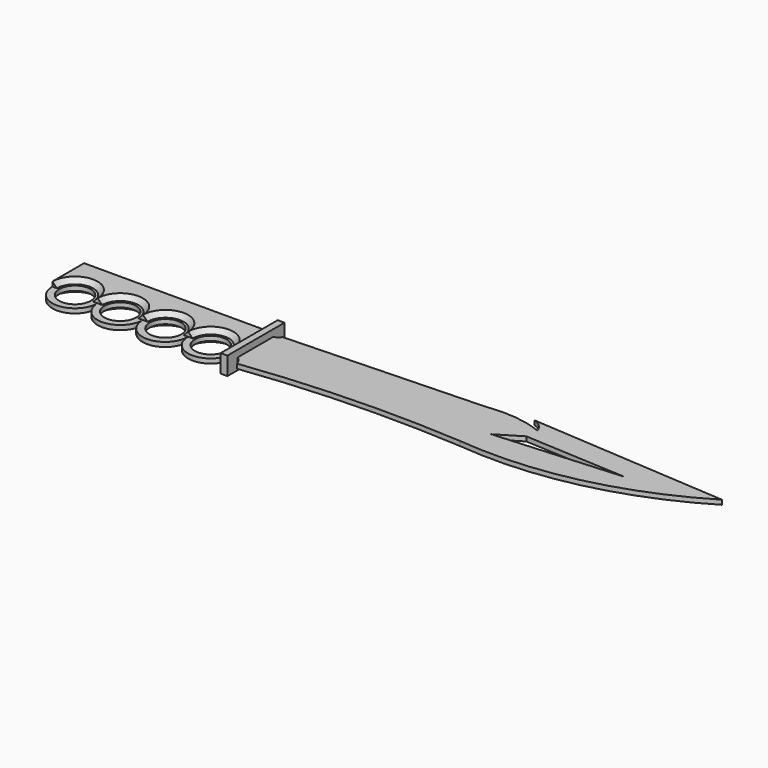
from build123d import *

# Parameters (mm, degrees)
F0_R          = 8.89
F1_DEPTH      = 2.54
F3_DEPTH      = 25.4
F5_DEPTH      = 2.54
F7_DEPTH      = 2.54
F8_T2_ANGLE   = 306.5001793885
F8_T4_ANGLE   = 306.5001793885
F8_T6_ANGLE   = 306.5001793885
F8_T8_ANGLE   = 306.5001793885
F8_2_T2_ANGLE = 306.5001793885
F8_2_T4_ANGLE = 306.5001793885
F8_2_T6_ANGLE = 306.5001793885
F8_2_T8_ANGLE = 306.5001793885
F10_DEPTH     = 3.81


# Not quite as in the source:
# - a fillet or chamfer that OpenCascade refuses, or shapes differently, is made with other operations: its cross-section is extruded or revolved along the edge and cut away or added


with BuildPart() as f1:
    # F0 (on Top) → F1 (new body)
    with BuildSketch(Plane.XY):
        with BuildLine():
            Line((0, 22.2569602452), (0, 0))
            ThreePointArc((0, 0), (4.5429449248, -2.2524889562), (7.2743112207, -6.5246890036))
            ThreePointArc((7.2743112207, -6.5246890036), (68.2558827077, -1.7283700883), (129.4168248237, -2.7752204279))
            ThreePointArc((129.4168248237, -2.7752204279), (193.990196572, 1.2229597331), (254, 25.4))
            Line((254, 25.4), (142.8799988323, 32.9367792524))
            Line((142.8799988323, 32.9367792524), (119.2322895651, 29.7860647099))
            ThreePointArc((119.2322895651, 29.7860647099), (116.0841208365, 29.5940132977), (112.9331847352, 29.4545436828))
            Line((112.9331847352, 29.4545436828), (7.2743112207, 25.6611633832))
            ThreePointArc((7.2743112207, 25.6611633832), (4.0157254245, 23.1501104869), (0, 22.2569602452))
        make_face()
        with BuildLine():
            ThreePointArc((-25.3981255835, -0.218189517), (-12.5909012159, -12.6995313872), (0, 0))
            Line((0, 0), (0, 22.2569602452))
            Line((0, 22.2569602452), (-34.8408528237, 22.2569602452))
            ThreePointArc((-34.8408528237, 22.2569602452), (-50.8, 21.91440634), (-66.7591471763, 22.2569602452))
            Line((-66.7591471763, 22.2569602452), (-101.6, 22.2569602452))
            Line((-101.6, 22.2569602452), (-101.6, 0))
            ThreePointArc((-101.6, 0), (-88.9, -12.7), (-76.2, 0))
            ThreePointArc((-76.2, 0), (-63.6090987841, -12.6995313872), (-50.8018744165, -0.218189517))
            ThreePointArc((-50.8018744165, -0.218189517), (-38.1, -12.9200800362), (-25.3981255835, -0.218189517))
        make_face()
        with Locations((-88.9, 0)):
            Circle(F0_R, mode=Mode.SUBTRACT)
        with Locations((-63.5, 0)):
            Circle(F0_R, mode=Mode.SUBTRACT)
        with BuildLine():
            ThreePointArc((-50.8, 0), (-50.8004686128, -0.1090987841), (-50.8018744165, -0.218189517))
            ThreePointArc((-50.8018744165, -0.218189517), (-50.8014057346, -0.1090907335), (-50.8, 0))
        make_face(mode=Mode.SUBTRACT)
        with Locations((-38.1, 0)):
            Circle(F0_R, mode=Mode.SUBTRACT)
        with BuildLine():
            ThreePointArc((-25.4, 0), (-25.3985942654, -0.1090907335), (-25.3981255835, -0.218189517))
            ThreePointArc((-25.3981255835, -0.218189517), (-25.3995313872, -0.1090987841), (-25.4, 0))
        make_face(mode=Mode.SUBTRACT)
        with Locations((-12.7, 0)):
            Circle(F0_R, mode=Mode.SUBTRACT)
        with BuildLine():
            ThreePointArc((-66.7591471763, 22.2569602452), (-50.8, 21.91440634), (-34.8408528237, 22.2569602452))
            Line((-34.8408528237, 22.2569602452), (-66.7591471763, 22.2569602452))
        make_face()
        with BuildLine():
            ThreePointArc((-50.8, 0), (-50.8014057346, -0.1090907335), (-50.8018744165, -0.218189517))
            ThreePointArc((-50.8018744165, -0.218189517), (-50.8004686128, -0.1090987841), (-50.8, 0))
        make_face()
        with BuildLine():
            ThreePointArc((-25.4, 0), (-25.3995313872, -0.1090987841), (-25.3981255835, -0.218189517))
            ThreePointArc((-25.3981255835, -0.218189517), (-25.3985942654, -0.1090907335), (-25.4, 0))
        make_face()
    extrude(amount=F1_DEPTH)

    # F2 (on face) → F3 (cut)
    with BuildSketch(Plane.XY.offset(2.54)):
        with BuildLine():
            ThreePointArc((119.2322895651, 29.7860647099), (134.7574672595, 29.9044998636), (149.8305946589, 26.1834785342))
            ThreePointArc((149.8305946589, 26.1834785342), (147.1610546869, 30.3894267459), (142.8799988323, 32.9367792524))
            Line((142.8799988323, 32.9367792524), (119.2322895651, 29.7860647099))
        make_face()
        Polygon((207.085609436, 15.6457461417), (149.4793444872, 18.8070647418), (136.1315399408, 10.7281366363), align=None)
    extrude(amount=-F3_DEPTH, mode=Mode.SUBTRACT)


with BuildPart() as f5:
    # F4 (on face) → F5 (new body)
    with BuildSketch(Plane.XY.offset(2.54)):
        with BuildLine():
            Line((0, 0), (0, 22.2569602452))
            Line((0, 22.2569602452), (-101.6, 22.2569602452))
            Line((-101.6, 22.2569602452), (-101.6, 0))
            Line((-101.6, 0), (-97.79, 0))
            ThreePointArc((-97.79, 0), (-88.9, 8.89), (-80.01, 0))
            Line((-80.01, 0), (-76.2, 0))
            Line((-76.2, 0), (-72.39, 0))
            ThreePointArc((-72.39, 0), (-63.5, 8.89), (-54.61, 0))
            Line((-54.61, 0), (-46.99, 0))
            ThreePointArc((-46.99, 0), (-38.1, 8.89), (-29.21, 0))
            Line((-29.21, 0), (-21.59, 0))
            ThreePointArc((-21.59, 0), (-12.7, 8.89), (-3.81, 0))
            Line((-3.81, 0), (0, 0))
        make_face()
    extrude(amount=F5_DEPTH)

    # F8: chamfer of 3.81 on 4 edges, made by hand

    # F8_s1 → F8_t2 (revolve, cut)
    with BuildSketch(Plane(origin=(-70.8899847432, 35.7313546731, 0), x_dir=(0, 0, 1), z_dir=(0.892979648, -0.4500970431, 0))):
        Polygon((5.08, 52.7136271329), (1.27, 48.9036271329), (5.08, 48.9036271329), align=None)
    revolve(axis=Axis((-88.9, 0, 5.08), (0, 0, -1)), revolution_arc=F8_T2_ANGLE, mode=Mode.SUBTRACT)

    # F8_s3 → F8_t4 (revolve, cut)
    with BuildSketch(Plane(origin=(-50.635703388, 25.5223961951, 0), x_dir=(0, 0, 1), z_dir=(0.892979648, -0.4500970431, 0))):
        Polygon((5.08, 41.2811622378), (1.27, 37.4711622378), (5.08, 37.4711622378), align=None)
    revolve(axis=Axis((-63.5, 0, 5.08), (0, 0, -1)), revolution_arc=F8_T4_ANGLE, mode=Mode.SUBTRACT)

    # F8_s5 → F8_t6 (revolve, cut)
    with BuildSketch(Plane(origin=(-30.3814220328, 15.3134377171, 0), x_dir=(0, 0, 1), z_dir=(0.892979648, -0.4500970431, 0))):
        Polygon((5.08, 29.8486973427), (1.27, 26.0386973427), (5.08, 26.0386973427), align=None)
    revolve(axis=Axis((-38.1, 0, 5.08), (0, 0, -1)), revolution_arc=F8_T6_ANGLE, mode=Mode.SUBTRACT)

    # F8_s7 → F8_t8 (revolve, cut)
    with BuildSketch(Plane(origin=(-10.1271406776, 5.104479239, 0), x_dir=(0, 0, 1), z_dir=(0.892979648, -0.4500970431, 0))):
        Polygon((5.08, 18.4162324476), (1.27, 14.6062324476), (5.08, 14.6062324476), align=None)
    revolve(axis=Axis((-12.7, 0, 5.08), (0, 0, -1)), revolution_arc=F8_T8_ANGLE, mode=Mode.SUBTRACT)


with BuildPart() as f7:
    # F6 (on face) → F7 (new body)
    with BuildSketch(Plane(origin=(0, 0, 0), x_dir=(1, 0, 0), z_dir=(0, 0, -1))):
        with BuildLine():
            Line((-101.6, -22.2569602452), (0, -22.2569602452))
            Line((0, -22.2569602452), (0, 0))
            Line((0, 0), (-3.81, 0))
            ThreePointArc((-3.81, 0), (-12.7, -8.89), (-21.59, 0))
            Line((-21.59, 0), (-29.21, 0))
            ThreePointArc((-29.21, 0), (-38.1, -8.89), (-46.99, 0))
            Line((-46.99, 0), (-54.61, 0))
            ThreePointArc((-54.61, 0), (-63.5, -8.89), (-72.39, 0))
            Line((-72.39, 0), (-76.2, 0))
            Line((-76.2, 0), (-80.01, 0))
            ThreePointArc((-80.01, 0), (-88.9, -8.89), (-97.79, 0))
            Line((-97.79, 0), (-101.6, 0))
            Line((-101.6, 0), (-101.6, -22.2569602452))
        make_face()
    extrude(amount=F7_DEPTH)

    # F8#2: chamfer of 3.81 on 4 edges, made by hand

    # F8_2_s1 → F8_2_t2 (revolve, cut)
    with BuildSketch(Plane(origin=(-30.3814220328, -15.3134377171, 0), x_dir=(0, 0, 1), z_dir=(-0.892979648, -0.4500970431, 0))):
        Polygon((-2.54, 4.4486973427), (1.27, 8.2586973427), (-2.54, 8.2586973427), align=None)
    revolve(axis=Axis((-38.1, 0, -2.54), (0, 0, 1)), revolution_arc=F8_2_T2_ANGLE, mode=Mode.SUBTRACT)

    # F8_2_s3 → F8_2_t4 (revolve, cut)
    with BuildSketch(Plane(origin=(-10.1271406776, -5.104479239, 0), x_dir=(0, 0, 1), z_dir=(-0.892979648, -0.4500970431, 0))):
        Polygon((-2.54, -6.9837675524), (1.27, -3.1737675524), (-2.54, -3.1737675524), align=None)
    revolve(axis=Axis((-12.7, 0, -2.54), (0, 0, 1)), revolution_arc=F8_2_T4_ANGLE, mode=Mode.SUBTRACT)

    # F8_2_s5 → F8_2_t6 (revolve, cut)
    with BuildSketch(Plane(origin=(-50.635703388, -25.5223961951, 0), x_dir=(0, 0, 1), z_dir=(-0.892979648, -0.4500970431, 0))):
        Polygon((-2.54, 15.8811622378), (1.27, 19.6911622378), (-2.54, 19.6911622378), align=None)
    revolve(axis=Axis((-63.5, 0, -2.54), (0, 0, 1)), revolution_arc=F8_2_T6_ANGLE, mode=Mode.SUBTRACT)

    # F8_2_s7 → F8_2_t8 (revolve, cut)
    with BuildSketch(Plane(origin=(-70.8899847432, -35.7313546731, 0), x_dir=(0, 0, 1), z_dir=(-0.892979648, -0.4500970431, 0))):
        Polygon((-2.54, 27.3136271329), (1.27, 31.1236271329), (-2.54, 31.1236271329), align=None)
    revolve(axis=Axis((-88.9, 0, -2.54), (0, 0, 1)), revolution_arc=F8_2_T8_ANGLE, mode=Mode.SUBTRACT)


with BuildPart() as f10:
    # F9 (on face) → F10 (new body)
    with BuildSketch(Plane.YZ):
        Polygon((0, -3.81), (22.2569602452, -3.81), (31.1469602452, -3.81), (31.1469602452, 6.35), (22.2569602452, 6.35), (0, 6.35), (-8.89, 6.35), (-8.89, -3.81), align=None)
        Polygon((22.2569602452, 2.54), (22.2569602452, 0), (22.2569602452, -2.54), (0, -2.54), (0, 0), (0, 2.54), align=None, mode=Mode.SUBTRACT)
    extrude(amount=F10_DEPTH)


solid = Compound([f1.part, f5.part, f7.part, f10.part])
